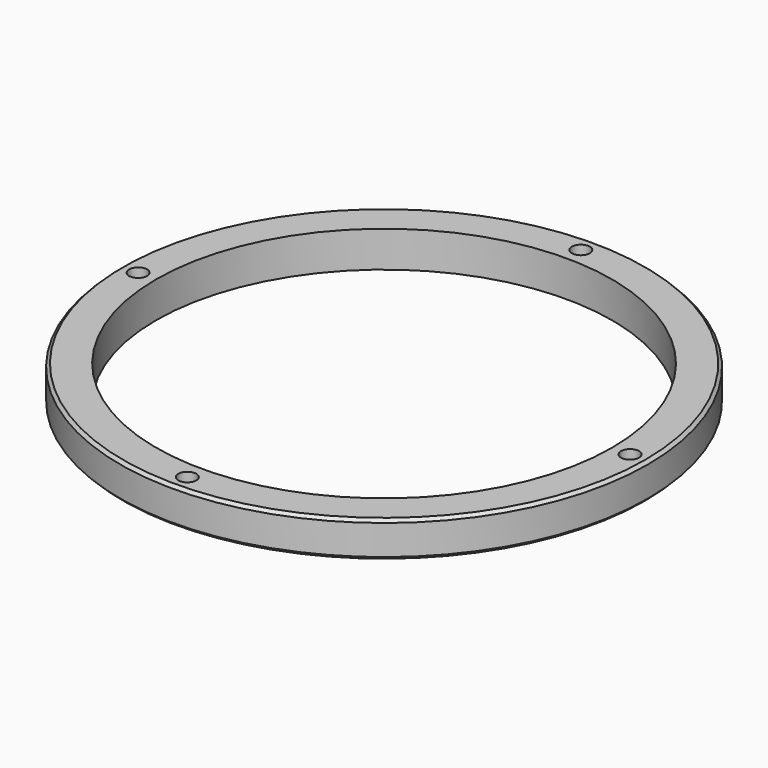
from build123d import *

# Parameters (mm, degrees)
F2_R      = 139.7
F3_DEPTH  = 19.05
F4_SIZE   = 1.5875
F5_R      = 120.65
F6_DEPTH  = 19.051
F7_R      = 0.79375
F8_DEPTH  = 19.051
F9_R      = 4.7625
F9_R_2    = 0.79375
F10_DEPTH = 15.875


# Not quite as in the source:
# - a variable given as a bare number and used for a length is read in inches; the dataset says mm whatever the document's units were


with BuildPart() as f3:
    # F2 (on Top) → F3 (new body)
    with BuildSketch(Plane.XY):
        Circle(F2_R)
    extrude(amount=F3_DEPTH)

    # F4
    f4_edges = [f3.edges().sort_by_distance(p)[0] for p in [
        (-139.7, 0, 19.05),
        (-139.7, 0, 0),
    ]]
    chamfer(f4_edges, length=F4_SIZE)

    # F5 (on face) → F6 (cut, through all)
    with BuildSketch(Plane(origin=(0, 0, 0), x_dir=(1, 0, 0), z_dir=(0, 0, -1))):
        Circle(F5_R)
    extrude(amount=-F6_DEPTH, mode=Mode.SUBTRACT)

    # F7 (on face) → F8 (cut, through all)
    with BuildSketch(Plane.XY.offset(19.05)):
        with Locations((0, 130.175)):
            Circle(F7_R)
        with Locations((130.175, 0)):
            Circle(F7_R)
        with Locations((0, -130.175)):
            Circle(F7_R)
        with Locations((-130.175, 0)):
            Circle(F7_R)
    extrude(amount=-F8_DEPTH, mode=Mode.SUBTRACT)

    # F9 (on face) → F10 (cut)
    with BuildSketch(Plane.XY.offset(19.05)):
        with Locations((0, 130.175)):
            Circle(F9_R)
        with Locations((0, 130.175)):
            Circle(F9_R_2, mode=Mode.SUBTRACT)
        with Locations((130.175, 0)):
            Circle(F9_R)
        with Locations((130.175, 0)):
            Circle(F9_R_2, mode=Mode.SUBTRACT)
        with Locations((-130.175, 0)):
            Circle(F9_R)
        with Locations((-130.175, 0)):
            Circle(F9_R_2, mode=Mode.SUBTRACT)
        with Locations((0, -130.175)):
            Circle(F9_R)
        with Locations((0, -130.175)):
            Circle(F9_R_2, mode=Mode.SUBTRACT)
    extrude(amount=-F10_DEPTH, mode=Mode.SUBTRACT)


solid = f3.part
